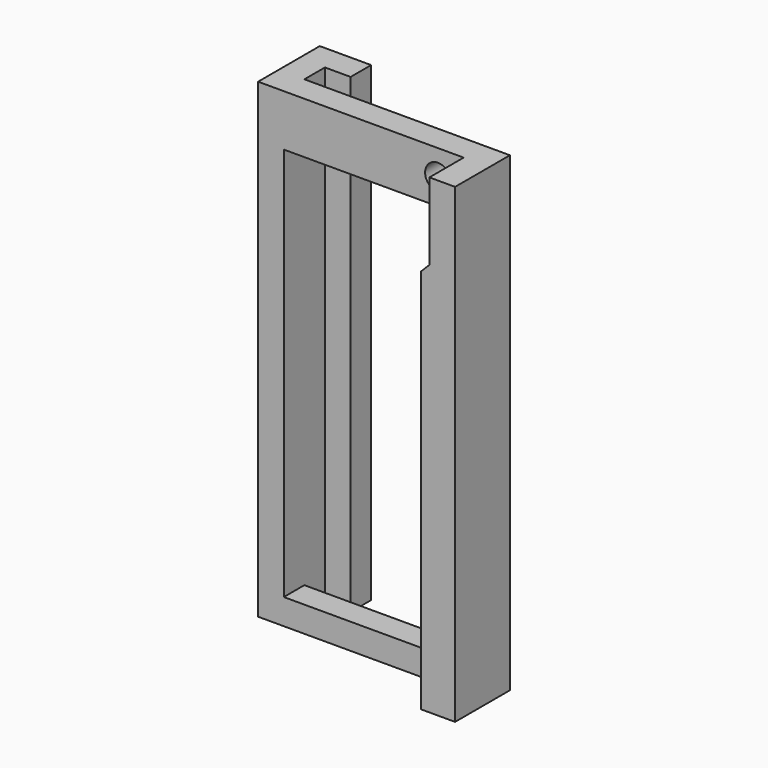
from build123d import *

# Parameters (mm, degrees)
F1_DEPTH = 55
F2_R     = 1.5
F2_W     = 21
F2_H     = 46
F3_DEPTH = 5
F4_W     = 3
F4_H     = 10
F5_DEPTH = 1
F6_SIZE  = 0.99999


# Not quite as in the source:
# - a fillet or chamfer is up to 0.001 mm smaller than in the source, because OpenCascade refuses the exact size


with BuildPart() as f1:
    # F0 (on Top) → F1 (new body)
    with BuildSketch(Plane.XY):
        Polygon((24, 0), (0, 0), (0, 2.9999995536), (3, 2.9999995536), (3, 5.9999995536), (-3, 5.9999995536), (-3, -3.0000002232), (21, -3.0000002232), (21, -5.0000002232), (20, -5.0000002232), (20, -8.0000002232), (24, -8.0000002232), align=None)
    extrude(amount=F1_DEPTH)

    # F2 (on face) → F3 (cut)
    with BuildSketch(Plane.XZ.offset(3.0000002232)):
        with Locations((18, 52)):
            Circle(F2_R)
        with Locations((10.5, 26)):
            Rectangle(F2_W, F2_H)
    extrude(amount=-F3_DEPTH, mode=Mode.SUBTRACT)

    # F4 (on face) → F5 (cut)
    with BuildSketch(Plane(origin=(20, 0, 0), x_dir=(0, -1, 0), z_dir=(-1, 0, 0))):
        with Locations((6.5000002232, 50)):
            Rectangle(F4_W, F4_H)
    extrude(amount=-F5_DEPTH, mode=Mode.SUBTRACT)

    # F6 (size 1 in the source; OpenCascade refuses exactly that, so slightly less here)
    f6_edges = [f1.edges().sort_by_distance(p)[0] for p in [
        (21, -6.5, 45),
    ]]
    chamfer(f6_edges, length=F6_SIZE)


solid = f1.part
